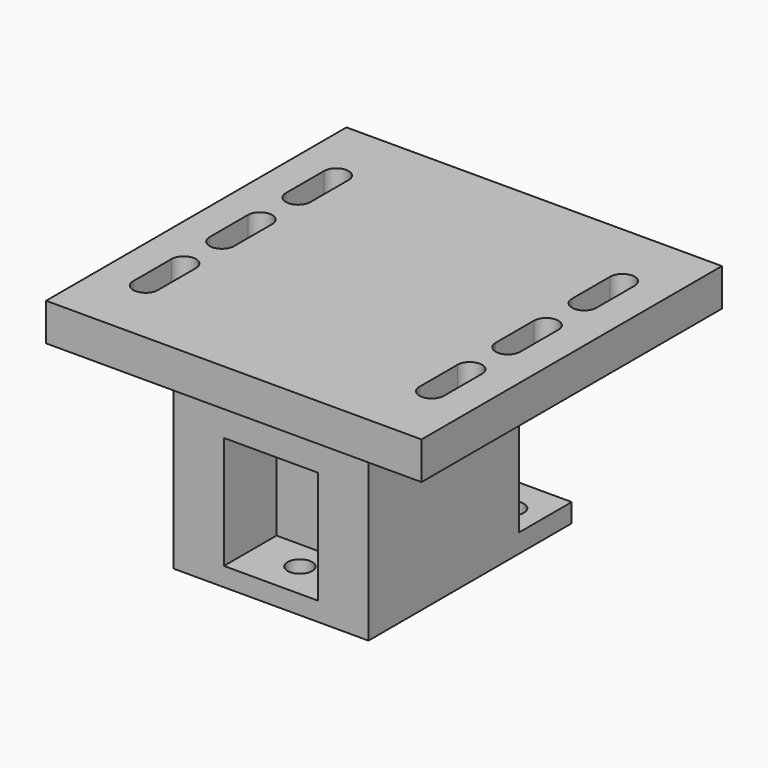
from build123d import *

# Parameters (mm, degrees)
F0_W      = 52
F0_H      = 67.66
F2_DEPTH  = 5
F1_R      = 3.265
F3_DEPTH  = 5
F4_W      = 52
F4_H      = 67.66
F5_DEPTH  = 30
F6_W      = 17.5
F6_H      = 17.5
F6_W_2    = 25
F7_DEPTH  = 30
F8_W      = 52
F8_H      = 67.66
F9_DEPTH  = 25
F10_W     = 100
F10_H     = 100
F11_DEPTH = 10
F13_DEPTH = 10


with BuildPart() as f2:
    # F0 (on Top) → F2 (new body)
    with BuildSketch(Plane.XY):
        with Locations((0, -3.83)):
            Rectangle(F0_W, F0_H)
    extrude(amount=F2_DEPTH)

    # F1 (on face) → F3 (cut)
    with BuildSketch(Plane.XY):
        with Locations((-18, 20)):
            Circle(F1_R)
        with Locations((18, 20)):
            Circle(F1_R)
        with Locations((0, -28)):
            Circle(F1_R)
    extrude(amount=F3_DEPTH, mode=Mode.SUBTRACT)

    # F4 (on face) → F5 (join)
    with BuildSketch(Plane.XY.offset(5)):
        with Locations((0, -3.83)):
            Rectangle(F4_W, F4_H)
    extrude(amount=F5_DEPTH)

    # F6 (on face) → F7 (cut)
    with BuildSketch(Plane.XY.offset(35)):
        with Locations((-17.25, 21.25)):
            Rectangle(F6_W, F6_H)
        with Locations((17.25, 21.25)):
            Rectangle(F6_W, F6_H)
        with Locations((0, -28.91)):
            Rectangle(F6_W_2, F6_H)
    extrude(amount=-F7_DEPTH, mode=Mode.SUBTRACT)

    # F8 (on face) → F9 (join)
    with BuildSketch(Plane.XY.offset(35)):
        with Locations((0, -3.83)):
            Rectangle(F8_W, F8_H)
    extrude(amount=F9_DEPTH)

    # F10 (on face) → F11 (join)
    with BuildSketch(Plane.XY.offset(60)):
        Rectangle(F10_W, F10_H)
    extrude(amount=-F11_DEPTH)

    # F12 (on face) → F13 (cut)
    with BuildSketch(Plane.XY.offset(60)):
        with BuildLine():
            Line((34.835, -6.35), (41.365, -6.35))
            ThreePointArc((41.365, -6.35), (38.1, -3.085), (34.835, -6.35))
        make_face()
        with BuildLine():
            ThreePointArc((34.835, -6.35), (38.1, -9.615), (41.365, -6.35))
            Line((41.365, -6.35), (34.835, -6.35))
        make_face()
        with BuildLine():
            ThreePointArc((34.835, -6.35), (38.1, -3.085), (41.365, -6.35))
            Line((41.365, -6.35), (41.365, 6.35))
            ThreePointArc((41.365, 6.35), (38.1, 3.085), (34.835, 6.35))
            Line((34.835, 6.35), (34.835, -6.35))
        make_face()
        with BuildLine():
            Line((34.835, 6.35), (41.365, 6.35))
            ThreePointArc((41.365, 6.35), (38.1, 9.615), (34.835, 6.35))
        make_face()
        with BuildLine():
            ThreePointArc((34.835, 6.35), (38.1, 3.085), (41.365, 6.35))
            Line((41.365, 6.35), (34.835, 6.35))
        make_face()
        with BuildLine():
            Line((34.835, -31.75), (41.365, -31.75))
            ThreePointArc((41.365, -31.75), (38.1, -28.485), (34.835, -31.75))
        make_face()
        with BuildLine():
            ThreePointArc((34.835, -31.75), (38.1, -35.015), (41.365, -31.75))
            Line((41.365, -31.75), (34.835, -31.75))
        make_face()
        with BuildLine():
            ThreePointArc((34.835, -31.75), (38.1, -28.485), (41.365, -31.75))
            Line((41.365, -31.75), (41.365, -19.05))
            ThreePointArc((41.365, -19.05), (38.1, -22.315), (34.835, -19.05))
            Line((34.835, -19.05), (34.835, -31.75))
        make_face()
        with BuildLine():
            Line((34.835, -19.05), (41.365, -19.05))
            ThreePointArc((41.365, -19.05), (38.1, -15.785), (34.835, -19.05))
        make_face()
        with BuildLine():
            ThreePointArc((34.835, -19.05), (38.1, -22.315), (41.365, -19.05))
            Line((41.365, -19.05), (34.835, -19.05))
        make_face()
        with BuildLine():
            ThreePointArc((34.835, 31.75), (38.1, 28.485), (41.365, 31.75))
            ThreePointArc((41.365, 31.75), (38.1, 35.015), (34.835, 31.75))
        make_face()
        with BuildLine():
            Line((41.365, 19.05), (41.365, 31.75))
            ThreePointArc((41.365, 31.75), (38.1, 28.485), (34.835, 31.75))
            Line((34.835, 31.75), (34.835, 19.05))
            ThreePointArc((34.835, 19.05), (38.1, 22.315), (41.365, 19.05))
        make_face()
        with BuildLine():
            ThreePointArc((34.835, 19.05), (38.1, 15.785), (41.365, 19.05))
            ThreePointArc((41.365, 19.05), (38.1, 22.315), (34.835, 19.05))
        make_face()
        with BuildLine():
            ThreePointArc((-41.365, -31.75), (-38.1, -35.015), (-34.835, -31.75))
            ThreePointArc((-34.835, -31.75), (-38.1, -28.485), (-41.365, -31.75))
        make_face()
        with BuildLine():
            ThreePointArc((-41.365, -31.75), (-38.1, -28.485), (-34.835, -31.75))
            Line((-34.835, -31.75), (-34.835, -19.05))
            ThreePointArc((-34.835, -19.05), (-38.1, -22.315), (-41.365, -19.05))
            Line((-41.365, -19.05), (-41.365, -31.75))
        make_face()
        with BuildLine():
            ThreePointArc((-41.365, -19.05), (-38.1, -22.315), (-34.835, -19.05))
            ThreePointArc((-34.835, -19.05), (-38.1, -15.785), (-41.365, -19.05))
        make_face()
        with BuildLine():
            ThreePointArc((-41.365, -6.35), (-38.1, -9.615), (-34.835, -6.35))
            ThreePointArc((-34.835, -6.35), (-38.1, -3.085), (-41.365, -6.35))
        make_face()
        with BuildLine():
            ThreePointArc((-41.365, -6.35), (-38.1, -3.085), (-34.835, -6.35))
            Line((-34.835, -6.35), (-34.835, 6.35))
            ThreePointArc((-34.835, 6.35), (-38.1, 3.085), (-41.365, 6.35))
            Line((-41.365, 6.35), (-41.365, -6.35))
        make_face()
        with BuildLine():
            ThreePointArc((-41.365, 6.35), (-38.1, 3.085), (-34.835, 6.35))
            ThreePointArc((-34.835, 6.35), (-38.1, 9.615), (-41.365, 6.35))
        make_face()
        with BuildLine():
            ThreePointArc((-41.365, 19.05), (-38.1, 15.785), (-34.835, 19.05))
            ThreePointArc((-34.835, 19.05), (-38.1, 22.315), (-41.365, 19.05))
        make_face()
        with BuildLine():
            ThreePointArc((-41.365, 19.05), (-38.1, 22.315), (-34.835, 19.05))
            Line((-34.835, 19.05), (-34.835, 31.75))
            ThreePointArc((-34.835, 31.75), (-38.1, 28.485), (-41.365, 31.75))
            Line((-41.365, 31.75), (-41.365, 19.05))
        make_face()
        with BuildLine():
            ThreePointArc((-41.365, 31.75), (-38.1, 28.485), (-34.835, 31.75))
            ThreePointArc((-34.835, 31.75), (-38.1, 35.015), (-41.365, 31.75))
        make_face()
    extrude(amount=-F13_DEPTH, mode=Mode.SUBTRACT)


solid = f2.part
